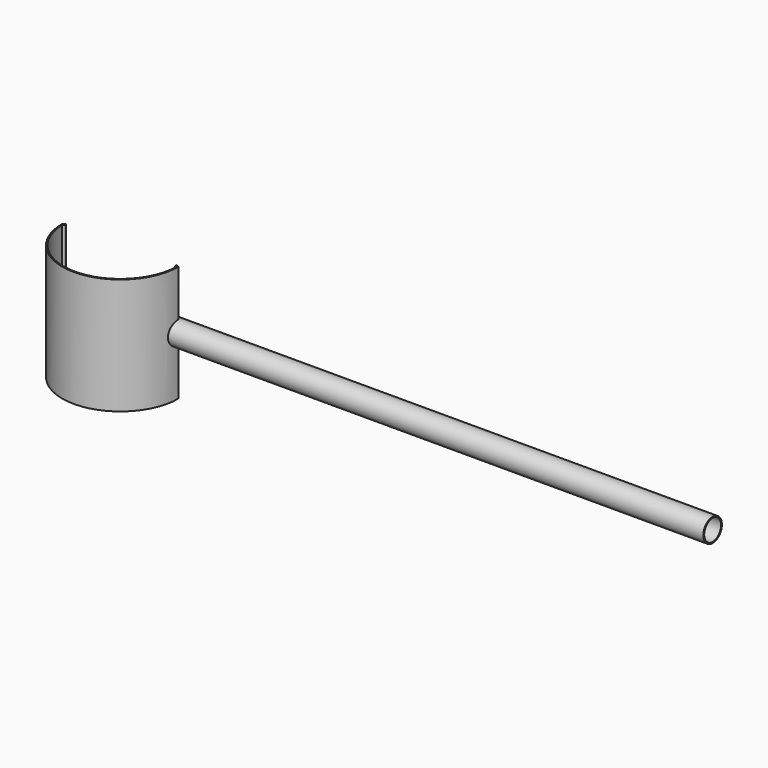
from build123d import *

# Parameters (mm, degrees)
F0_R      = 25
F1_DEPTH  = 50
F2_R      = 24.5
F3_DEPTH  = 49
F4_W      = 133.0040432513
F4_H      = 80.2016193047
F5_DEPTH  = 25
F7_DEPTH  = 49
F8_W      = 90.9072607756
F8_H      = 76.9354877993
F9_DEPTH  = 25
F11_R     = 5.0048176475
F11_R_2   = 4.4964097491
F12_DEPTH = 255
F13_DEPTH = 22
F14_R     = 4.5351415883
F15_DEPTH = 500


with BuildPart() as f1:
    # F0 (on Top) → F1 (new body)
    with BuildSketch(Plane.XY):
        Circle(F0_R)
    extrude(amount=F1_DEPTH)

    # F2 (on face) → F3 (cut)
    with BuildSketch(Plane.XY.offset(50)):
        Circle(F2_R)
    extrude(amount=-F3_DEPTH, mode=Mode.SUBTRACT)

    # F4 (on Front) → F5 (cut)
    with BuildSketch(Plane.XZ):
        with Locations((-6.1693545431, 24.7681471519)):
            Rectangle(F4_W, F4_H)
    extrude(amount=-F5_DEPTH, mode=Mode.SUBTRACT)

    # F6 (on face) → F7 (join)
    with BuildSketch(Plane.XY.offset(1)):
        with BuildLine():
            ThreePointArc((-23.7997439297, 0.2099188306), (-23.7849922899, 0.2579040005), (-23.7800096296, 0.307857584))
            ThreePointArc((-23.7800096296, 0.307857584), (-23.7800491855, 0.3123303341), (-23.780167841, 0.3168016851))
            ThreePointArc((-23.780167841, 0.3168016851), (-23.8565770485, 0.4891434991), (-24.0309707308, 0.5607459532))
            ThreePointArc((-24.0309707308, 0.5607459532), (-23.8896091672, 0.4023027599), (-23.7997439297, 0.2099188306))
        make_face()
        with BuildLine():
            ThreePointArc((-23.780167841, 0.3168016851), (-23.7800491855, 0.3123303341), (-23.7800096296, 0.307857584))
            ThreePointArc((-23.7800096296, 0.307857584), (-23.7849922899, 0.2579040005), (-23.7997439297, 0.2099188306))
            ThreePointArc((-23.7997439297, 0.2099188306), (-23.780898653, 0.1315968548), (-23.77078537, 0.0516769082))
            Line((-23.77078537, 0.0516769082), (-23.780167841, 0.3168016851))
        make_face()
        with BuildLine():
            ThreePointArc((-23.77078537, 0.0516769082), (-23.780898653, 0.1315968548), (-23.7997439297, 0.2099188306))
            ThreePointArc((-23.7997439297, 0.2099188306), (-24.1447977278, 0.0810616911), (-24.2525015897, 0.4332919626))
            Line((-24.2525015897, 0.4332919626), (-24.5, 0))
            Line((-24.5, 0), (-23.7689565817, 0))
            Line((-23.7689565817, 0), (-23.77078537, 0.0516769082))
        make_face()
        with BuildLine():
            ThreePointArc((-24.2525015897, 0.4332919626), (-24.1447977278, 0.0810616911), (-23.7997439297, 0.2099188306))
            ThreePointArc((-23.7997439297, 0.2099188306), (-23.8896091672, 0.4023027599), (-24.0309707308, 0.5607459532))
            ThreePointArc((-24.0309707308, 0.5607459532), (-24.1590214746, 0.5270629802), (-24.2525015897, 0.4332919626))
        make_face()
        with BuildLine():
            ThreePointArc((-24.5, 0), (-24.4972731927, -0.3655217092), (-24.489093378, -0.7309620544))
            ThreePointArc((-24.489093378, -0.7309620544), (-23.9792324445, -0.5130551945), (-23.7689565817, 0))
            Line((-23.7689565817, 0), (-24.5, 0))
        make_face()
    extrude(amount=F7_DEPTH)

    # F8 (on Right) → F9 (cut)
    with BuildSketch(Plane.YZ):
        with Locations((-10.7056461275, 28.0342758633)):
            Rectangle(F8_W, F8_H)
    extrude(amount=F9_DEPTH, mode=Mode.SUBTRACT)

    # F10: F1 across face


with BuildPart() as f1_1:
    add(f1.part)
    add(f1.part.mirror(Plane(origin=(0, -18.5631313131, 12.8737373737), x_dir=(0, 1, 0), z_dir=(1, 0, 0))))

    # F11 (on Right) → F12 (join)
    with BuildSketch(Plane.YZ):
        with Locations((0, 25.0316294775)):
            Circle(F11_R)
        with Locations((0, 25.0316294775)):
            Circle(F11_R_2, mode=Mode.SUBTRACT)
    extrude(amount=F12_DEPTH)

    # F11 (on Right) → F13 (cut)
    with BuildSketch(Plane.YZ):
        with Locations((0, 25.0316294775)):
            Circle(F11_R)
        with Locations((0, 25.0316294775)):
            Circle(F11_R_2, mode=Mode.SUBTRACT)
    extrude(amount=F13_DEPTH, mode=Mode.SUBTRACT)

    # F14 (on Right) → F15 (cut)
    with BuildSketch(Plane.YZ):
        with Locations((0, 25.0294525176)):
            Circle(F14_R)
    extrude(amount=F15_DEPTH, mode=Mode.SUBTRACT)


solid = f1_1.part
